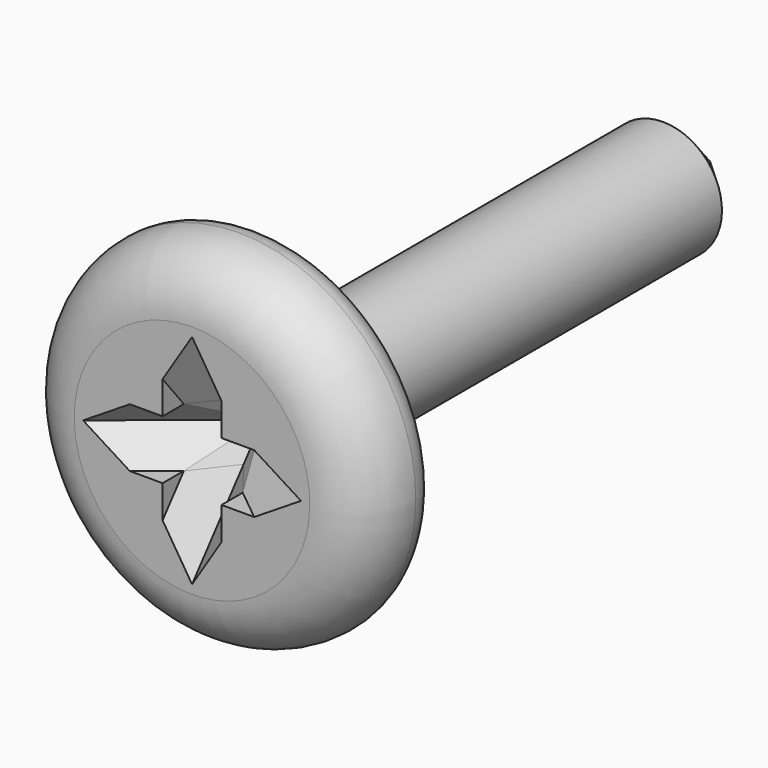
from build123d import *

# Parameters (mm, degrees)
F2_SIZE      = 1
F4_DEPTH     = 0.5
F5_T4_DEPTH  = 4.9533840607
F5_T10_DEPTH = 4.9533840607
F5_T16_DEPTH = 4.9533840607
F5_T22_DEPTH = 4.9533840607
F7_DEPTH     = 0.5
F8_T4_DEPTH  = 4.9533840607
F8_T10_DEPTH = 4.9533840607
F8_T16_DEPTH = 4.9533840607
F8_T22_DEPTH = 4.9533840607
F8_T28_DEPTH = 4.9533840607
F8_T34_DEPTH = 4.9533840607
F8_T40_DEPTH = 4.9533840607
F8_T46_DEPTH = 4.9533840607


# Not quite as in the source:
# - a fillet or chamfer that OpenCascade refuses, or shapes differently, is made with other operations: its cross-section is extruded or revolved along the edge and cut away or added


with BuildPart() as f1:
    # F0 (on Right) → F1 (revolve)
    with BuildSketch(Plane.YZ):
        with BuildLine():
            Line((0, 2), (0, 0))
            Line((0, 0), (11, 0))
            Line((11, 0), (11, 1))
            Line((11, 1), (1.5, 1))
            Line((1.5, 1), (1.5, 2.5))
            ThreePointArc((1.5, 2.5), (1.3535533906, 2.8535533906), (1, 3))
            ThreePointArc((1, 3), (0.2928932188, 2.7071067812), (0, 2))
        make_face()
    revolve(axis=Axis((0, -4.3078260496, 0), (0, -1, 0)))

    # F2
    f2_edges = [f1.edges().sort_by_distance(p)[0] for p in [
        (0, 11, -1),
    ]]
    chamfer(f2_edges, length=F2_SIZE)

    # F3 (on Right) → F4 (cut, symmetric)
    with BuildSketch(Plane.YZ):
        Polygon((1.5, 0), (0, 1.85), (0, -1.85), align=None)
    extrude(amount=F4_DEPTH, both=True, mode=Mode.SUBTRACT)

    # F5: chamfer of 0.5 on 4 edges, made by hand


with BuildPart() as f5_tool2:
    # F5_s3 → F5_t4 (new body)
    with BuildSketch(Plane(origin=(0, -1.7148497309, -2.1149813348), x_dir=(1, 0, 0), z_dir=(0, 0.6298019584, 0.7767557487))):
        Polygon((0, 1.1651336231), (0.5, 0.6651336231), (0.5, 1.1651336231), align=None)
    extrude(amount=F5_T4_DEPTH)

    split(bisect_by=Plane.XZ, keep=Keep.BOTTOM)

    split(bisect_by=Plane(origin=(0, 0.9050242398, 0.7338034376), x_dir=(1, 0, 0), z_dir=(0, -0.7767557487, -0.6298019584)), keep=Keep.TOP)


with BuildPart() as f1_1:
    add(f1.part)

    # F5_t1: union F5_tool2
    add(f5_tool2.part)


with BuildPart() as f5_tool8:
    # F5_s9 → F5_t10 (new body)
    with BuildSketch(Plane(origin=(0, -1.7148497309, -2.1149813348), x_dir=(1, 0, 0), z_dir=(0, 0.6298019584, 0.7767557487))):
        Polygon((-0.5, 0.6651336231), (0, 1.1651336231), (-0.5, 1.1651336231), align=None)
    extrude(amount=F5_T10_DEPTH)

    split(bisect_by=Plane.XZ, keep=Keep.BOTTOM)

    split(bisect_by=Plane(origin=(0, 0.9050242398, 0.7338034376), x_dir=(1, 0, 0), z_dir=(0, -0.7767557487, -0.6298019584)), keep=Keep.TOP)


with BuildPart() as f1_2:
    add(f1_1.part)

    # F5_t7: union F5_tool8
    add(f5_tool8.part)


with BuildPart() as f5_tool14:
    # F5_s15 → F5_t16 (new body)
    with BuildSketch(Plane(origin=(0, 1.4048012514, -1.73258821), x_dir=(1, 0, 0), z_dir=(0, -0.6298019584, 0.7767557487))):
        Polygon((-0.5, 0.6651336231), (0, 1.1651336231), (-0.5, 1.1651336231), align=None)
    extrude(amount=F5_T16_DEPTH)

    split(bisect_by=Plane.XZ, keep=Keep.BOTTOM)

    split(bisect_by=Plane(origin=(0, 0.9050242398, -0.7338034376), x_dir=(1, 0, 0), z_dir=(0, -0.7767557487, 0.6298019584)), keep=Keep.TOP)


with BuildPart() as f1_3:
    add(f1_2.part)

    # F5_t13: union F5_tool14
    add(f5_tool14.part)


with BuildPart() as f5_tool20:
    # F5_s21 → F5_t22 (new body)
    with BuildSketch(Plane(origin=(0, 1.4048012514, -1.73258821), x_dir=(1, 0, 0), z_dir=(0, -0.6298019584, 0.7767557487))):
        Polygon((0.5, 0.6651336231), (0, 1.1651336231), (0.5, 1.1651336231), align=None)
    extrude(amount=F5_T22_DEPTH)

    split(bisect_by=Plane.XZ, keep=Keep.BOTTOM)

    split(bisect_by=Plane(origin=(0, 0.9050242398, -0.7338034376), x_dir=(1, 0, 0), z_dir=(0, -0.7767557487, 0.6298019584)), keep=Keep.TOP)


with BuildPart() as f1_4:
    add(f1_3.part)

    # F5_t19: union F5_tool20
    add(f5_tool20.part)

    # F6 (on Top) → F7 (cut, symmetric)
    with BuildSketch(Plane.XY):
        Polygon((0, 1.5), (-1.85, 0), (1.85, 0), align=None)
    extrude(amount=F7_DEPTH, both=True, mode=Mode.SUBTRACT)

    # F8: chamfer of 0.5 on 4 edges, made by hand


with BuildPart() as f8_tool2:
    # F8_s3 → F8_t4 (new body)
    with BuildSketch(Plane(origin=(2.1149813348, -1.7148497309, 0), x_dir=(0, 0, 1), z_dir=(-0.7767557487, 0.6298019584, 0))):
        Polygon((0, 1.1651336231), (-0.5, 0.6651336231), (-0.5, 1.1651336231), align=None)
    extrude(amount=F8_T4_DEPTH)

    split(bisect_by=Plane.XZ, keep=Keep.BOTTOM)

    split(bisect_by=Plane(origin=(0.5825668116, 0.4525121199, -0.3669017188), x_dir=(-0.6134375783, 0.7897432099, 0), z_dir=(0.7071067812, 0.5492492572, -0.4453372356)), keep=Keep.TOP)


with BuildPart() as f1_5:
    add(f1_4.part)

    # F8_t1: union F8_tool2
    add(f8_tool2.part)


with BuildPart() as f8_tool8:
    # F8_s9 → F8_t10 (new body)
    with BuildSketch(Plane(origin=(2.1149813348, -1.7148497309, 0), x_dir=(0, 0, 1), z_dir=(-0.7767557487, 0.6298019584, 0))):
        Polygon((0, 1.1651336231), (-0.5, 0.6651336231), (-0.5, 1.1651336231), align=None)
    extrude(amount=F8_T10_DEPTH)

    split(bisect_by=Plane(origin=(-0.5825668116, 0.4525121199, -0.3669017188), x_dir=(-0.6134375783, -0.7897432099, 0), z_dir=(-0.7071067812, 0.5492492572, -0.4453372356)), keep=Keep.TOP)

    split(bisect_by=Plane(origin=(-0.7338034376, 0.9050242398, 0), x_dir=(0, 0, 1), z_dir=(0.6298019584, -0.7767557487, 0)), keep=Keep.TOP)


with BuildPart() as f1_6:
    add(f1_5.part)

    # F8_t7: union F8_tool8
    add(f8_tool8.part)


with BuildPart() as f8_tool14:
    # F8_s15 → F8_t16 (new body)
    with BuildSketch(Plane(origin=(1.73258821, 1.4048012514, 0), x_dir=(0, 0, 1), z_dir=(-0.7767557487, -0.6298019584, 0))):
        Polygon((-0.5, 0.6651336231), (0, 1.1651336231), (-0.5, 1.1651336231), align=None)
    extrude(amount=F8_T16_DEPTH)

    split(bisect_by=Plane(origin=(0.7338034376, 0.9050242398, 0), x_dir=(0, 0, 1), z_dir=(-0.6298019584, -0.7767557487, 0)), keep=Keep.TOP)

    split(bisect_by=Plane(origin=(0.5825668116, 0.4525121199, -0.3669017188), x_dir=(-0.6134375783, 0.7897432099, 0), z_dir=(0.7071067812, 0.5492492572, -0.4453372356)), keep=Keep.TOP)


with BuildPart() as f1_7:
    add(f1_6.part)

    # F8_t13: union F8_tool14
    add(f8_tool14.part)


with BuildPart() as f8_tool20:
    # F8_s21 → F8_t22 (new body)
    with BuildSketch(Plane(origin=(1.73258821, 1.4048012514, 0), x_dir=(0, 0, 1), z_dir=(-0.7767557487, -0.6298019584, 0))):
        Polygon((-0.5, 0.6651336231), (0, 1.1651336231), (-0.5, 1.1651336231), align=None)
    extrude(amount=F8_T22_DEPTH)

    split(bisect_by=Plane.XZ, keep=Keep.BOTTOM)

    split(bisect_by=Plane(origin=(-0.5825668116, 0.4525121199, -0.3669017188), x_dir=(-0.6134375783, -0.7897432099, 0), z_dir=(-0.7071067812, 0.5492492572, -0.4453372356)), keep=Keep.TOP)


with BuildPart() as f1_8:
    add(f1_7.part)

    # F8_t19: union F8_tool20
    add(f8_tool20.part)


with BuildPart() as f8_tool26:
    # F8_s27 → F8_t28 (new body)
    with BuildSketch(Plane(origin=(2.1149813348, -1.7148497309, 0), x_dir=(0, 0, 1), z_dir=(-0.7767557487, 0.6298019584, 0))):
        Polygon((0, 1.1651336231), (0.5, 0.6651336231), (0.5, 1.1651336231), align=None)
    extrude(amount=F8_T28_DEPTH)

    split(bisect_by=Plane.XZ, keep=Keep.BOTTOM)

    split(bisect_by=Plane(origin=(0.5825668116, 0.4525121199, 0.3669017188), x_dir=(-0.6134375783, 0.7897432099, 0), z_dir=(0.7071067812, 0.5492492572, 0.4453372356)), keep=Keep.TOP)


with BuildPart() as f1_9:
    add(f1_8.part)

    # F8_t25: union F8_tool26
    add(f8_tool26.part)


with BuildPart() as f8_tool32:
    # F8_s33 → F8_t34 (new body)
    with BuildSketch(Plane(origin=(2.1149813348, -1.7148497309, 0), x_dir=(0, 0, 1), z_dir=(-0.7767557487, 0.6298019584, 0))):
        Polygon((0, 1.1651336231), (0.5, 0.6651336231), (0.5, 1.1651336231), align=None)
    extrude(amount=F8_T34_DEPTH)

    split(bisect_by=Plane(origin=(-0.5825668116, 0.4525121199, 0.3669017188), x_dir=(-0.6134375783, -0.7897432099, 0), z_dir=(-0.7071067812, 0.5492492572, 0.4453372356)), keep=Keep.TOP)

    split(bisect_by=Plane(origin=(-0.7338034376, 0.9050242398, 0), x_dir=(0, 0, 1), z_dir=(0.6298019584, -0.7767557487, 0)), keep=Keep.TOP)


with BuildPart() as f1_10:
    add(f1_9.part)

    # F8_t31: union F8_tool32
    add(f8_tool32.part)


with BuildPart() as f8_tool38:
    # F8_s39 → F8_t40 (new body)
    with BuildSketch(Plane(origin=(1.73258821, 1.4048012514, 0), x_dir=(0, 0, 1), z_dir=(-0.7767557487, -0.6298019584, 0))):
        Polygon((0, 1.1651336231), (0.5, 0.6651336231), (0.5, 1.1651336231), align=None)
    extrude(amount=F8_T40_DEPTH)

    split(bisect_by=Plane(origin=(0.5825668116, 0.4525121199, 0.3669017188), x_dir=(-0.6134375783, 0.7897432099, 0), z_dir=(0.7071067812, 0.5492492572, 0.4453372356)), keep=Keep.TOP)

    split(bisect_by=Plane(origin=(0.7338034376, 0.9050242398, 0), x_dir=(0, 0, 1), z_dir=(-0.6298019584, -0.7767557487, 0)), keep=Keep.TOP)


with BuildPart() as f1_11:
    add(f1_10.part)

    # F8_t37: union F8_tool38
    add(f8_tool38.part)


with BuildPart() as f8_tool44:
    # F8_s45 → F8_t46 (new body)
    with BuildSketch(Plane(origin=(1.73258821, 1.4048012514, 0), x_dir=(0, 0, 1), z_dir=(-0.7767557487, -0.6298019584, 0))):
        Polygon((0, 1.1651336231), (0.5, 0.6651336231), (0.5, 1.1651336231), align=None)
    extrude(amount=F8_T46_DEPTH)

    split(bisect_by=Plane.XZ, keep=Keep.BOTTOM)

    split(bisect_by=Plane(origin=(-0.5825668116, 0.4525121199, 0.3669017188), x_dir=(-0.6134375783, -0.7897432099, 0), z_dir=(-0.7071067812, 0.5492492572, 0.4453372356)), keep=Keep.TOP)


with BuildPart() as f1_12:
    add(f1_11.part)

    # F8_t43: union F8_tool44
    add(f8_tool44.part)


solid = f1_12.part
